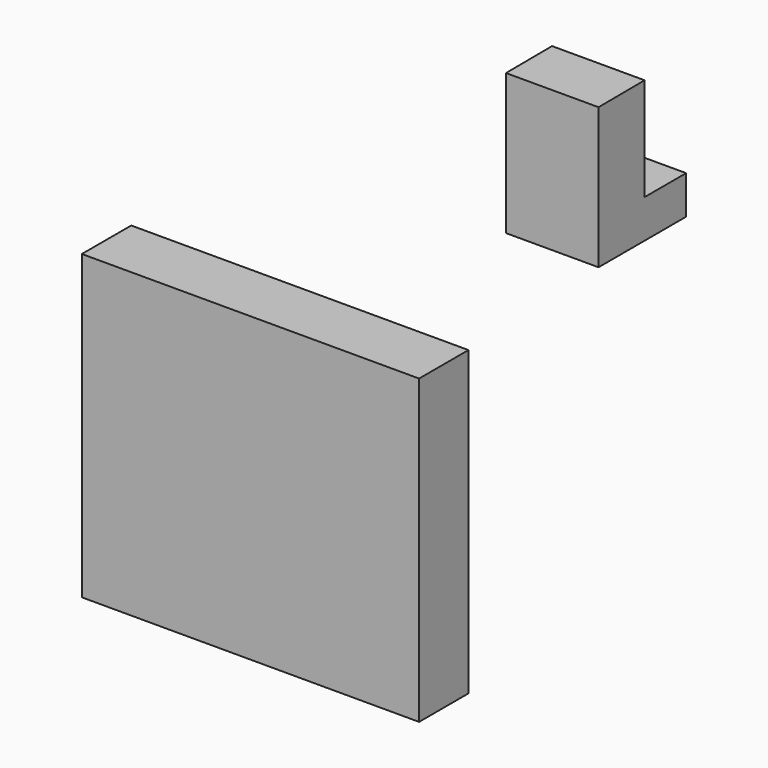
from build123d import *

# Parameters (mm, degrees)
F0_W     = 69.4220066071
F0_H     = 62.2280314565
F3_DEPTH = 12.7
F5_DEPTH = 19.05


# Not quite as in the source:
# - the program builds the solid bodies; features that only make, move or delete a surface that nothing else refers to are left out


with BuildPart() as f3:
    # F0 (on Front) → F3 (new body)
    with BuildSketch(Plane.XZ):
        with Locations((-5.8741644025, 9.6652619541)):
            Rectangle(F0_W, F0_H)
    extrude(amount=F3_DEPTH)


with BuildPart() as f5:
    # F4 (on Right) → F5 (new body)
    with BuildSketch(Plane.YZ):
        Polygon((57.5543679297, 63.0933269858), (45.7089096308, 63.025817275), (45.7089096308, 34.0147763491), (68.2484209538, 34.0147763491), (68.2484209538, 41.9166460633), (57.5543679297, 41.9166460633), align=None)
    extrude(amount=F5_DEPTH)


solid = Compound([f3.part, f5.part])
